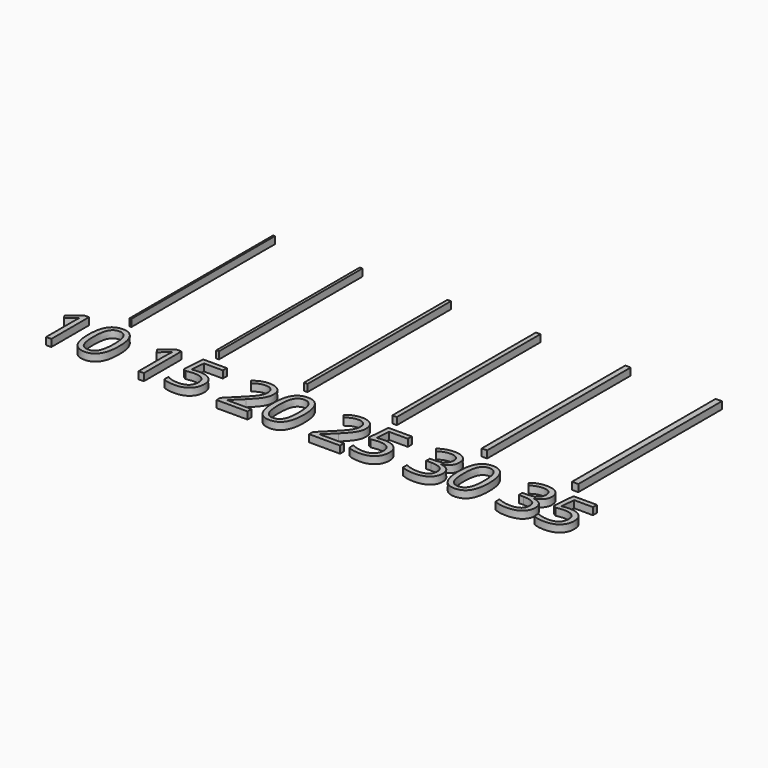
from build123d import *

# Parameters (mm, degrees)
F0_W         = 0.254
F0_H         = 25.4
F0_W_2       = 0.381
F0_W_3       = 0.508
F0_W_4       = 0.635
F0_W_5       = 0.762
F0_W_6       = 0.889
F0_TEXT_SIZE = 9.3300172183
F1_DEPTH     = 1.016


# Not quite as in the source:
# - Text() gives the source's letters only with a copy of the font that has no kerning and outlines rounded to 1/6400 em; it was checked with that copy


with BuildPart() as f1:
    # F0 (on Top) → F1 (new body)
    with BuildSketch(Plane.XY):
        with Locations((-31.0515, 12.7)):
            Rectangle(F0_W, F0_H)
        with Locations((-18.7198, 12.7)):
            Rectangle(F0_W_2, F0_H)
        with Locations((-6.2611, 12.7)):
            Rectangle(F0_W_3, F0_H)
        with Locations((6.3246, 12.7)):
            Rectangle(F0_W_4, F0_H)
        with Locations((19.0373, 12.7)):
            Rectangle(F0_W_5, F0_H)
        with Locations((31.877, 12.7)):
            Rectangle(F0_W_6, F0_H)
        with Locations((-38.1, -9.2576123972)):
            Text('10 15 20 25 30 35', F0_TEXT_SIZE, font='Open Sans', text_align=(TextAlign.LEFT, TextAlign.BOTTOM))
    extrude(amount=F1_DEPTH)


solid = f1.part
